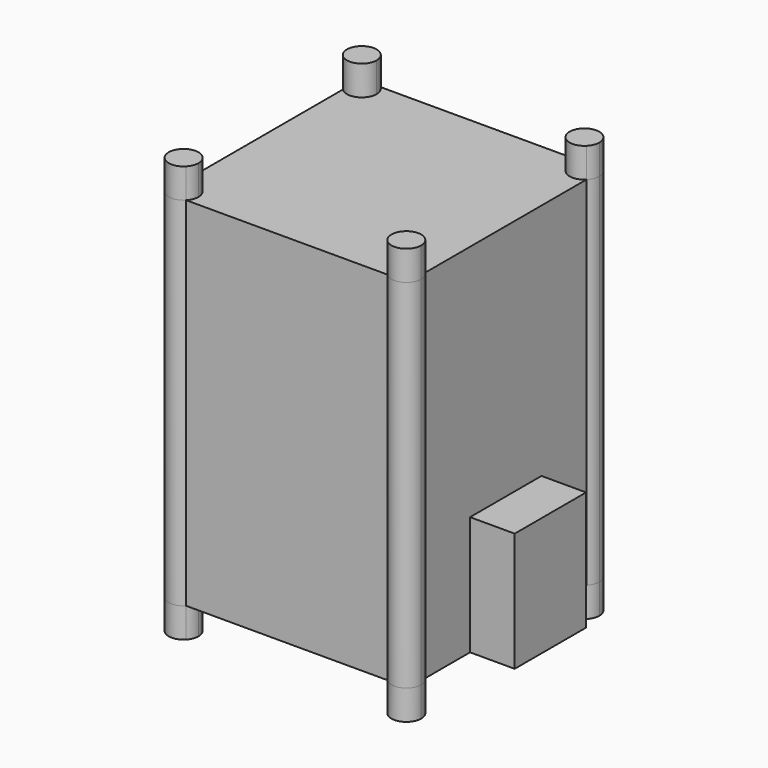
from build123d import *

# Parameters (mm, degrees)
F1_DEPTH = 82.55
F2_DEPTH = 76.2
F0_W     = 9.525
F0_H     = 19.05
F3_DEPTH = 25.4


# Not quite as in the source:
# - a feature of the source that left no trace in its solid (it failed there, or was rolled back) is left out
# - a pattern or mirror of a feature is missing from the dataset's text; its kind, count and spacing are read off the source's solid


with BuildPart() as f1:
    # F0 (on Top) → F1 (new body)
    with BuildSketch(Plane.XY):
        with BuildLine():
            ThreePointArc((-20.197500676, 18.3455366127), (-16.7326156752, 17.6181000932), (-14.7552827986, 20.5548919915))
            ThreePointArc((-14.7552827986, 20.5548919915), (-15.044803813, 21.8783314962), (-15.8604748841, 22.9599946804))
            ThreePointArc((-15.8604748841, 22.9599946804), (-20.234431152, 22.7256124785), (-20.197500676, 18.3455366127))
        make_face()
    extrude(amount=F1_DEPTH)

    # F1_copies: F1 across plane


with BuildPart() as f1b:
    # F0 (on Top) → F1, piece 2 (new body)
    with BuildSketch(Plane.XY):
        with BuildLine():
            ThreePointArc((32.7525223778, 20.5548919915), (30.9204110591, 23.4204148874), (27.5505643884, 22.9599946804))
            ThreePointArc((27.5505643884, 22.9599946804), (27.2638489298, 18.4265931888), (31.8045291463, 18.2994790273))
            ThreePointArc((31.8045291463, 18.2994790273), (32.5058902534, 19.3316198625), (32.7525223778, 20.5548919915))
        make_face()
    extrude(amount=F1_DEPTH)

    # F1_2_copies: F1b across plane


with BuildPart() as f1c:
    # F0 (on Top) → F1, piece 3 (new body)
    with BuildSketch(Plane.XY):
        with BuildLine():
            ThreePointArc((32.7651335661, -26.9655103104), (32.5151222308, -25.7316713922), (31.8045291463, -24.6924786227))
            ThreePointArc((31.8045291463, -24.6924786227), (27.3600452383, -24.7185591863), (27.3112643614, -29.1628519118))
            ThreePointArc((27.3112643614, -29.1628519118), (30.7800389767, -29.9054507611), (32.7651335661, -26.9655103104))
        make_face()
    extrude(amount=F1_DEPTH)

    # F1_3_copies: F1c across plane


with BuildPart() as f1d:
    # F0 (on Top) → F1, piece 4 (new body)
    with BuildSketch(Plane.XY):
        with BuildLine():
            ThreePointArc((-14.7564191649, -26.9655103104), (-16.7335847801, -24.0295514846), (-20.197500676, -24.7577854871))
            ThreePointArc((-20.197500676, -24.7577854871), (-20.1273922452, -29.2431839447), (-15.6421652409, -29.1628519118))
            ThreePointArc((-15.6421652409, -29.1628519118), (-14.9861867967, -28.150083675), (-14.7564191649, -26.9655103104))
        make_face()
    extrude(amount=F1_DEPTH)

    # F1_4_copies: F1d across plane


with BuildPart() as f1_1:
    add(f1.part)
    add(f1.part.mirror(Plane(origin=(0, 0, 38.1), x_dir=(-1, 0, 0), z_dir=(0, 0, -1))))



with BuildPart() as f1b_1:
    add(f1b.part)
    add(f1b.part.mirror(Plane(origin=(0, 0, 38.1), x_dir=(-1, 0, 0), z_dir=(0, 0, -1))))


with BuildPart() as f1c_1:
    add(f1c.part)
    add(f1c.part.mirror(Plane(origin=(0, 0, 38.1), x_dir=(-1, 0, 0), z_dir=(0, 0, -1))))


with BuildPart() as f1d_1:
    add(f1d.part)
    add(f1d.part.mirror(Plane(origin=(0, 0, 38.1), x_dir=(-1, 0, 0), z_dir=(0, 0, -1))))


with BuildPart() as f1_2:
    add(f1_1.part)

    add(f1b_1.part)  # F2 merges F1b

    add(f1c_1.part)  # F2 merges F1c

    add(f1d_1.part)  # F2 merges F1d
    # F0 (on Top) → F2 (join)
    with BuildSketch(Plane.XY):
        with BuildLine():
            ThreePointArc((-15.8604748841, 22.9599946804), (-15.044803813, 21.8783314962), (-14.7552827986, 20.5548919915))
            ThreePointArc((-14.7552827986, 20.5548919915), (-16.7326156752, 17.6181000932), (-20.197500676, 18.3455366127))
            Line((-20.197500676, 18.3455366127), (-20.197500676, 6.3188755628))
            Line((-20.197500676, 6.3188755628), (-20.197500676, -12.7311244372))
            Line((-20.197500676, -12.7311244372), (-20.197500676, -24.7577854871))
            ThreePointArc((-20.197500676, -24.7577854871), (-16.7335847801, -24.0295514846), (-14.7564191649, -26.9655103104))
            ThreePointArc((-14.7564191649, -26.9655103104), (-14.9861867967, -28.150083675), (-15.6421652409, -29.1628519118))
            Line((-15.6421652409, -29.1628519118), (27.3112643614, -29.1628519118))
            ThreePointArc((27.3112643614, -29.1628519118), (27.3600452383, -24.7185591863), (31.8045291463, -24.6924786227))
            Line((31.8045291463, -24.6924786227), (31.8045291463, -12.7214997977))
            Line((31.8045291463, -12.7214997977), (31.8045291463, 6.3285002023))
            Line((31.8045291463, 6.3285002023), (31.8045291463, 18.2994790273))
            ThreePointArc((31.8045291463, 18.2994790273), (27.2638489298, 18.4265931888), (27.5505643884, 22.9599946804))
            Line((27.5505643884, 22.9599946804), (-15.8604748841, 22.9599946804))
        make_face()
    extrude(amount=F2_DEPTH)

    # F0 (on Top) → F3 (join)
    with BuildSketch(Plane.XY):
        with Locations((-24.960000676, -3.2061244372)):
            Rectangle(F0_W, F0_H)
        with Locations((36.5670291463, -3.1964997977)):
            Rectangle(F0_W, F0_H)
    extrude(amount=F3_DEPTH)


solid = f1_2.part
